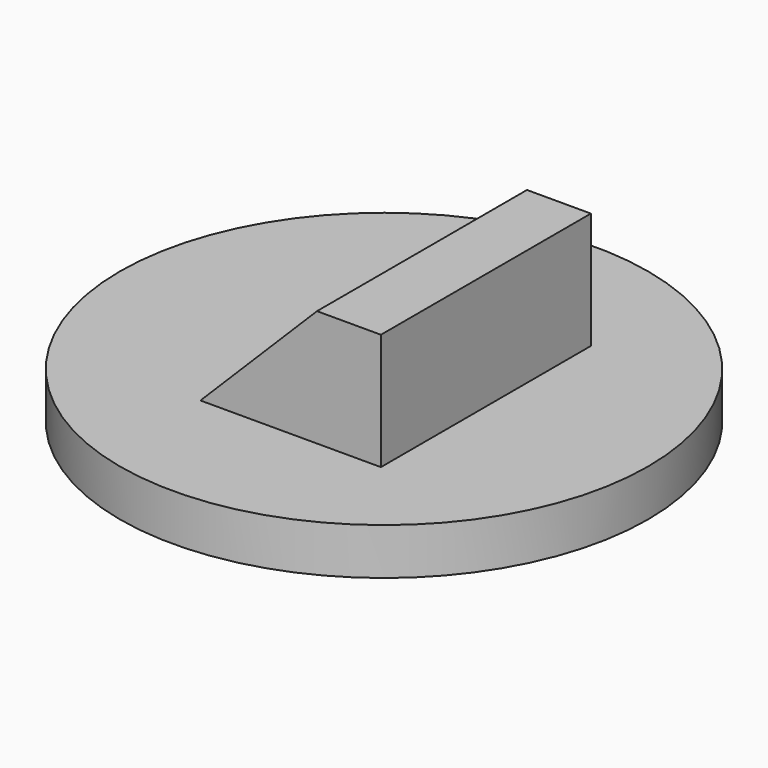
from build123d import *

# Parameters (mm, degrees)
F0_R        = 56.6549127416
F1_DEPTH    = 10
F2_W        = 43.7059700489
F2_H        = 56.300342083
F3_DEPTH    = 25
F4_T4_DEPTH = 210.6013213609


# Not quite as in the source:
# - a fillet or chamfer that OpenCascade refuses, or shapes differently, is made with other operations: its cross-section is extruded or revolved along the edge and cut away or added


with BuildPart() as f1:
    # F0 (on Top) → F1 (new body)
    with BuildSketch(Plane.XY):
        Circle(F0_R)
    extrude(amount=F1_DEPTH)

    # F2 (on face) → F3 (join)
    with BuildSketch(Plane.XY.offset(10)):
        Rectangle(F2_W, F2_H)
    extrude(amount=F3_DEPTH)

    # F4: chamfer of 30 on 1 edges, made by hand


with BuildPart() as f4_tool2:
    # F4_s3 → F4_t4 (new body)
    with BuildSketch(Plane.XZ.offset(-105.3006606805)):
        Polygon((-21.8529850245, 5), (8.1470149755, 35), (-21.8529850245, 35), align=None)
    extrude(amount=F4_T4_DEPTH)

    split(bisect_by=Plane.XY.offset(10), keep=Keep.TOP)


with BuildPart() as f1_1:
    add(f1.part)

    # F4_t1: cut F4_tool2
    add(f4_tool2.part, mode=Mode.SUBTRACT)


solid = f1_1.part
